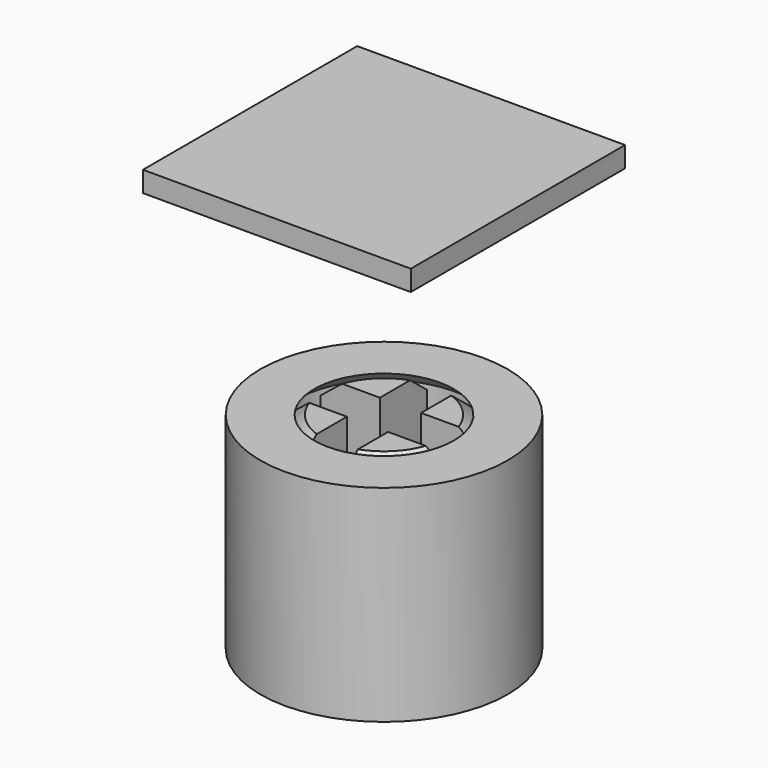
from build123d import *

# Parameters (mm, degrees)
F3_R      = 6
F4_DEPTH  = 10
F5_OFFSET = 0.25
F6_START  = 2
F2_W      = 2
F2_H      = 2
F6_DEPTH  = 8
F8_W      = 13
F8_H      = 13
F9_DEPTH  = 1


with BuildPart() as f1:
    # F0 (on Front) → F1 (revolve)
    with BuildSketch(Plane.XZ):
        Polygon((3, 10), (0, 10), (0, 0), (4, 0), (4, 6), (5, 7), (4, 8), (4, 9.1609003688), align=None)
    revolve(axis=Axis((0, 0, 5), (0, 0, 1)))


with BuildPart() as f4:
    # F3 (on Top) → F4 (new body, through all)
    with BuildSketch(Plane.XY):
        Circle(F3_R)
    extrude(amount=F4_DEPTH)

    # F5: cut F1, made larger all round first
    f5_tool = offset(f1.part, amount=F5_OFFSET, kind=Kind.INTERSECTION, mode=Mode.PRIVATE)
    add(f5_tool, mode=Mode.SUBTRACT)


with BuildPart() as f1_1:
    add(f1.part)

    # F2 (on Top) → F6 (cut)
    with BuildSketch(Plane.XY.offset(F6_START)):
        with BuildLine():
            ThreePointArc((0, -5), (0.50254481, -4.974680765), (1, -4.8989794856))
            Line((1, -4.8989794856), (1, -3.8729833462))
            ThreePointArc((1, -3.8729833462), (0, -4), (-1, -3.8729833462))
            Line((-1, -3.8729833462), (-1, -4.8989794856))
            ThreePointArc((-1, -4.8989794856), (-0.50254481, -4.974680765), (0, -5))
        make_face()
        with BuildLine():
            ThreePointArc((4.8989794856, -1), (4.974680765, -0.50254481), (5, 0))
            ThreePointArc((5, 0), (4.974680765, 0.50254481), (4.8989794856, 1))
            Line((4.8989794856, 1), (3.8729833462, 1))
            ThreePointArc((3.8729833462, 1), (3.9681187851, 0.5040171699), (4, 0))
            ThreePointArc((4, 0), (3.9681187851, -0.5040171699), (3.8729833462, -1))
            Line((3.8729833462, -1), (4.8989794856, -1))
        make_face()
        with BuildLine():
            Line((-3.8729833462, 1), (-4.8989794856, 1))
            ThreePointArc((-4.8989794856, 1), (-4.974680765, 0.50254481), (-5, 0))
            ThreePointArc((-5, 0), (-4.974680765, -0.50254481), (-4.8989794856, -1))
            Line((-4.8989794856, -1), (-3.8729833462, -1))
            ThreePointArc((-3.8729833462, -1), (-4, 0), (-3.8729833462, 1))
        make_face()
        with BuildLine():
            ThreePointArc((-1, -3.8729833462), (0, -4), (1, -3.8729833462))
            Line((1, -3.8729833462), (1, -2.8284271247))
            ThreePointArc((1, -2.8284271247), (0, -3), (-1, -2.8284271247))
            Line((-1, -2.8284271247), (-1, -3.8729833462))
        make_face()
        with BuildLine():
            ThreePointArc((-1, -2.8284271247), (0, -3), (1, -2.8284271247))
            Line((1, -2.8284271247), (1, -1))
            Line((1, -1), (-1, -1))
            Line((-1, -1), (-1, -2.8284271247))
        make_face()
        Rectangle(F2_W, F2_H)
        with BuildLine():
            Line((-1, -1), (-1, 1))
            Line((-1, 1), (-2.8284271247, 1))
            ThreePointArc((-2.8284271247, 1), (-3, 0), (-2.8284271247, -1))
            Line((-2.8284271247, -1), (-1, -1))
        make_face()
        with BuildLine():
            Line((-2.8284271247, 1), (-3.8729833462, 1))
            ThreePointArc((-3.8729833462, 1), (-4, 0), (-3.8729833462, -1))
            Line((-3.8729833462, -1), (-2.8284271247, -1))
            ThreePointArc((-2.8284271247, -1), (-3, 0), (-2.8284271247, 1))
        make_face()
        with BuildLine():
            ThreePointArc((3, 0), (2.956795679, 0.5073059362), (2.8284271247, 1))
            Line((2.8284271247, 1), (1, 1))
            Line((1, 1), (1, -1))
            Line((1, -1), (2.8284271247, -1))
            ThreePointArc((2.8284271247, -1), (2.956795679, -0.5073059362), (3, 0))
        make_face()
        with BuildLine():
            ThreePointArc((4, 0), (3.9681187851, 0.5040171699), (3.8729833462, 1))
            Line((3.8729833462, 1), (2.8284271247, 1))
            ThreePointArc((2.8284271247, 1), (2.956795679, 0.5073059362), (3, 0))
            ThreePointArc((3, 0), (2.956795679, -0.5073059362), (2.8284271247, -1))
            Line((2.8284271247, -1), (3.8729833462, -1))
            ThreePointArc((3.8729833462, -1), (3.9681187851, -0.5040171699), (4, 0))
        make_face()
        with BuildLine():
            Line((1, 1), (1, 2.8284271247))
            ThreePointArc((1, 2.8284271247), (0, 3), (-1, 2.8284271247))
            Line((-1, 2.8284271247), (-1, 1))
            Line((-1, 1), (1, 1))
        make_face()
        with BuildLine():
            Line((1, 2.8284271247), (1, 3.8729833462))
            ThreePointArc((1, 3.8729833462), (0, 4), (-1, 3.8729833462))
            Line((-1, 3.8729833462), (-1, 2.8284271247))
            ThreePointArc((-1, 2.8284271247), (0, 3), (1, 2.8284271247))
        make_face()
        with BuildLine():
            Line((1, 3.8729833462), (1, 4.8989794856))
            ThreePointArc((1, 4.8989794856), (0.50254481, 4.974680765), (0, 5))
            ThreePointArc((0, 5), (-0.50254481, 4.974680765), (-1, 4.8989794856))
            Line((-1, 4.8989794856), (-1, 3.8729833462))
            ThreePointArc((-1, 3.8729833462), (0, 4), (1, 3.8729833462))
        make_face()
    extrude(amount=F6_DEPTH, mode=Mode.SUBTRACT)


with BuildPart() as f9:
    # F8 (on offset) → F9 (new body)
    with BuildSketch(Plane.XY.offset(20)):
        Rectangle(F8_W, F8_H)
    extrude(amount=F9_DEPTH)


solid = Compound([f4.part, f1_1.part, f9.part])
